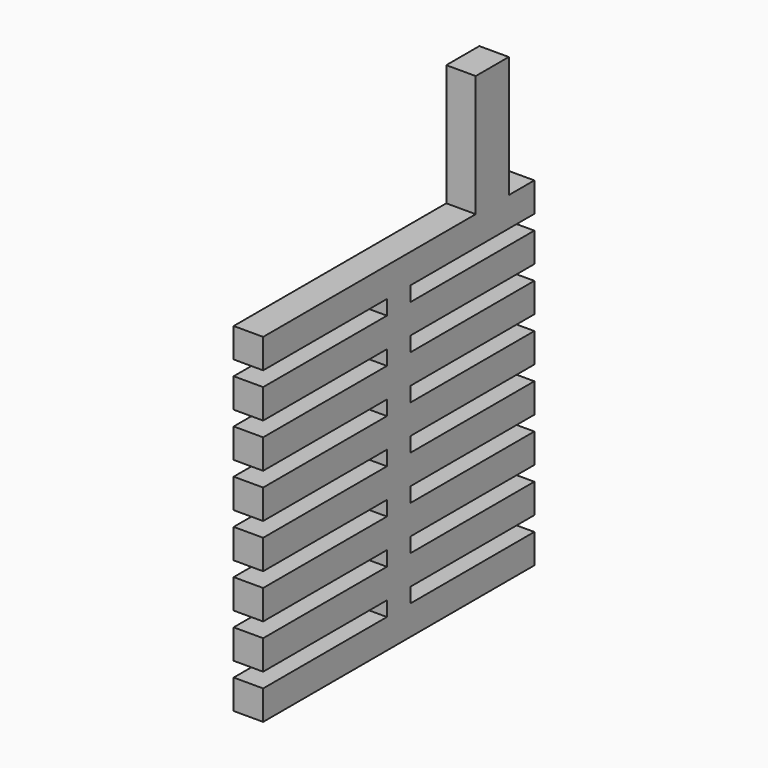
from build123d import *

# Parameters (mm, degrees)
F1_DEPTH = 1


# Not quite as in the source:
# - a feature names something its author has since deleted; it is built from what else it names


with BuildPart() as f1:
    # F0 (on Right) → F1 (new body)
    with BuildSketch(Plane.YZ):
        Polygon((0, 0.75), (0, 0), (0, -0.25), (11.5, -0.25), (11.5, 0), (11.5, 0.75), (11.25, 0.75), (6.25, 0.75), (6.25, 1.25), (11.25, 1.25), (11.5, 1.25), (11.5, 2.25), (11.25, 2.25), (6.25, 2.25), (6.25, 2.75), (11.25, 2.75), (11.5, 2.75), (11.5, 3.75), (11.25, 3.75), (6.25, 3.75), (6.25, 4.25), (11.25, 4.25), (11.5, 4.25), (11.5, 5.25), (11.25, 5.25), (6.25, 5.25), (6.25, 5.75), (11.25, 5.75), (11.5, 5.75), (11.5, 6.75), (11.25, 6.75), (6.25, 6.75), (6.25, 7.25), (11.25, 7.25), (11.5, 7.25), (11.5, 8.25), (11.25, 8.25), (6.25, 8.25), (6.25, 8.75), (11.25, 8.75), (11.5, 8.75), (11.5, 9.75), (11.25, 9.75), (6.25, 9.75), (6.25, 10.25), (11.25, 10.25), (11.5, 10.25), (11.5, 11.25), (10.4177193716, 11.25), (10.4177193716, 15.3758693486), (9.0160202235, 15.3758693486), (9.0160202235, 11.25), (0, 11.25), (0, 10.25), (0.25, 10.25), (5.25, 10.25), (5.25, 9.75), (0.25, 9.75), (0, 9.75), (0, 8.75), (0.25, 8.75), (5.25, 8.75), (5.25, 8.25), (0.25, 8.25), (0, 8.25), (0, 7.25), (0.25, 7.25), (5.25, 7.25), (5.25, 6.75), (0.25, 6.75), (0, 6.75), (0, 5.75), (0.25, 5.75), (5.25, 5.75), (5.25, 5.25), (0.25, 5.25), (0, 5.25), (0, 4.25), (0.25, 4.25), (5.25, 4.25), (5.25, 3.75), (0.25, 3.75), (0, 3.75), (0, 2.75), (0.25, 2.75), (5.25, 2.75), (5.25, 2.25), (0.25, 2.25), (0, 2.25), (0, 1.25), (0.25, 1.25), (5.25, 1.25), (5.25, 0.75), (0.25, 0.75), align=None)
    extrude(amount=F1_DEPTH)


solid = f1.part
